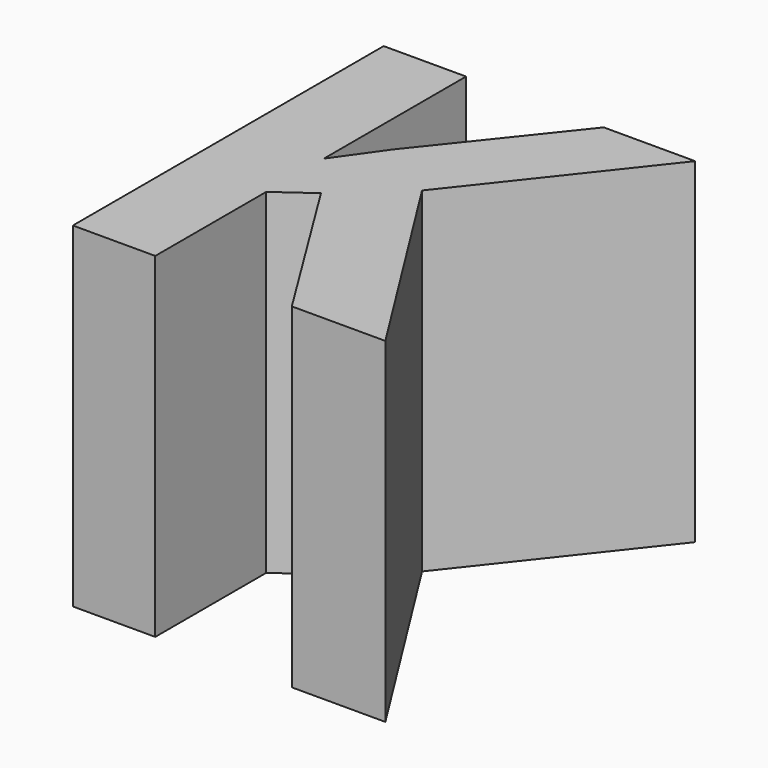
from build123d import *

# Parameters (mm, degrees)
F1_TEXT_SIZE = 41.212940899
F2_DEPTH     = 25.4


# Not quite as in the source:
# - Text() gives the source's letters only with a copy of the font that has no kerning and outlines rounded to 1/6400 em; it was checked with that copy


with BuildPart() as f2:
    # F1 (on offset) → F2 (new body)
    with BuildSketch(Plane.XY.offset(25.4)):
        with Locations((-19.332613796, 0)):
            Text('K', F1_TEXT_SIZE, font='Open Sans', font_style=FontStyle.BOLD, text_align=(TextAlign.LEFT, TextAlign.BOTTOM))
    extrude(amount=F2_DEPTH)


solid = f2.part
